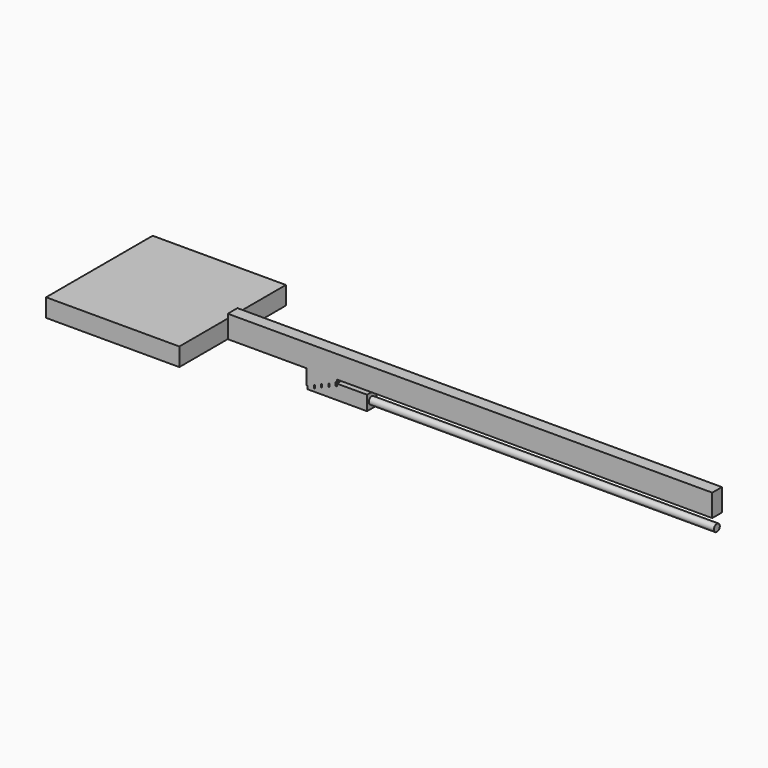
from build123d import *

# Parameters (mm, degrees)
F2_W      = 203.2
F2_H      = 5.08
F3_DEPTH  = 9.398
F0_W      = 12.7
F0_H      = 5.08
F12_DEPTH = 7.62
F11_W     = 0.508
F11_H     = 1.524
F11_H_2   = 1.27
F13_DEPTH = 2.54
F15_W     = 55.88
F15_H     = 55.88
F16_DEPTH = 7.62
F17_DEPTH = 6.096
F18_R     = 1.524


# Not quite as in the source:
# - a feature names something its author has since deleted; it is built from what else it names


with BuildPart() as f3:
    # F2 (on offset) → F3 (new body)
    with BuildSketch(Plane.XY.offset(7.62)):
        with Locations((43.18, 4.064)):
            Rectangle(F2_W, F2_H)
    extrude(amount=F3_DEPTH)

    # F0 (on Top) → F12 (join)
    with BuildSketch(Plane.XY):
        with Locations((-19.05, 4.064)):
            Rectangle(F0_W, F0_H)
    extrude(amount=F12_DEPTH)

    # F11 (on offset) → F13 (cut, symmetric)
    with BuildSketch(Plane.XZ.offset(-4.064)):
        with Locations((-12.954, 5.842)):
            Rectangle(F11_W, F11_H)
        with Locations((-25.146, 0.635)):
            Rectangle(F11_W, F11_H_2)
        with Locations((-19.05, 3.175)):
            Rectangle(F11_W, F11_H_2)
        with Locations((-16.002, 4.445)):
            Rectangle(F11_W, F11_H_2)
        with Locations((-22.098, 1.905)):
            Rectangle(F11_W, F11_H_2)
    extrude(amount=F13_DEPTH, both=True, mode=Mode.SUBTRACT)

    # F15 (on offset) → F16 (join)
    with BuildSketch(Plane.XY.offset(7.62)):
        with Locations((-86.36, 4.064)):
            Rectangle(F15_W, F15_H)
    extrude(amount=F16_DEPTH)

    # F0 (on Top) → F17 (join)
    with BuildSketch(Plane.XY):
        Polygon((-6.35, 1.524), (0, 1.524), (0, 6.604), (-12.7, 6.604), (-12.7, 1.524), align=None)
    extrude(amount=F17_DEPTH)

    # F21: sweep along a path in F20
    with BuildLine(Plane.XZ.offset(-3.9624)) as f21_path:
        Line((0, 3.048), (144.78, 3.048))
    # F18 (on Right) → F21 (sweep)
    with BuildSketch(Plane.YZ):
        with Locations((3.9624, 3.048)):
            Circle(F18_R)
    sweep(path=f21_path.line)


solid = f3.part
